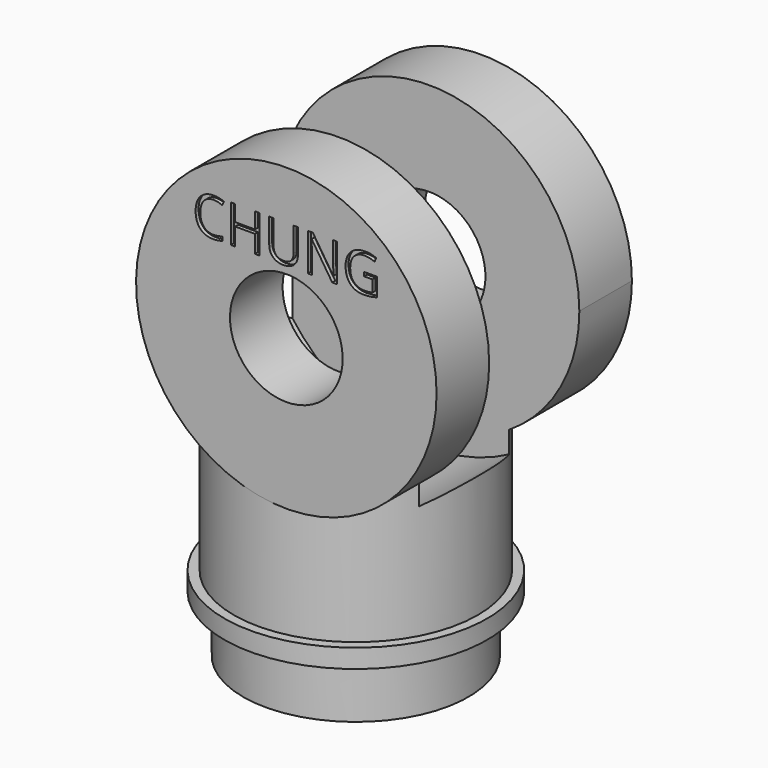
from build123d import *

# Parameters (mm, degrees)
F2_R          = 32.5
F3_DEPTH      = 70
F4_R          = 40
F5_DEPTH      = 32.5
F7_R          = 45
F8_DEPTH      = 15
F9_R          = 15
F10_DEPTH     = 67.501
F11_TEXT_SIZE = 14.0043763676
F12_DEPTH     = 1


# Not quite as in the source:
# - a feature names something its author has since deleted; it is built from what else it names
# - Text() gives the source's letters only with a copy of the font that has no kerning and outlines rounded to 1/6400 em; it was checked with that copy


with BuildPart() as f1:
    # F0 (on Front) → F1 (revolve)
    with BuildSketch(Plane.XZ):
        Polygon((-30, 0), (0, 0), (0, 20), (-35, 20), (-35, 15), (-30, 15), (-30, 14), (-31, 14), (-31, 13), (-30, 13), align=None)
    revolve(axis=Axis((0, 0, 10), (0, 0, 1)))

    # F2 (on face) → F3 (join)
    with BuildSketch(Plane.XY.offset(20)):
        Circle(F2_R)
    extrude(amount=F3_DEPTH)

    # F4 (on Front) → F5 (join, symmetric)
    with BuildSketch(Plane.XZ):
        with Locations((7.5, 90)):
            Circle(F4_R)
    extrude(amount=F5_DEPTH, both=True)

    # F7 (on Front) → F8 (cut, symmetric)
    with BuildSketch(Plane.XZ):
        with Locations((7.5, 90)):
            Circle(F7_R)
    extrude(amount=F8_DEPTH, both=True, mode=Mode.SUBTRACT)

    # F9 (on face) → F10 (cut, through all)
    with BuildSketch(Plane(origin=(0, 32.5, 0), x_dir=(-1, 0, 0), z_dir=(0, 1, 0))):
        with Locations((-7.5, 90)):
            Circle(F9_R)
    extrude(amount=-F10_DEPTH, mode=Mode.SUBTRACT)

    # F11 (on face) → F12 (cut)
    with BuildSketch(Plane.XZ.offset(32.5)):
        with Locations((-17.5, 107)):
            Text('CHUNG', F11_TEXT_SIZE, font='Open Sans', text_align=(TextAlign.LEFT, TextAlign.BOTTOM))
    extrude(amount=-F12_DEPTH, mode=Mode.SUBTRACT)


solid = f1.part
